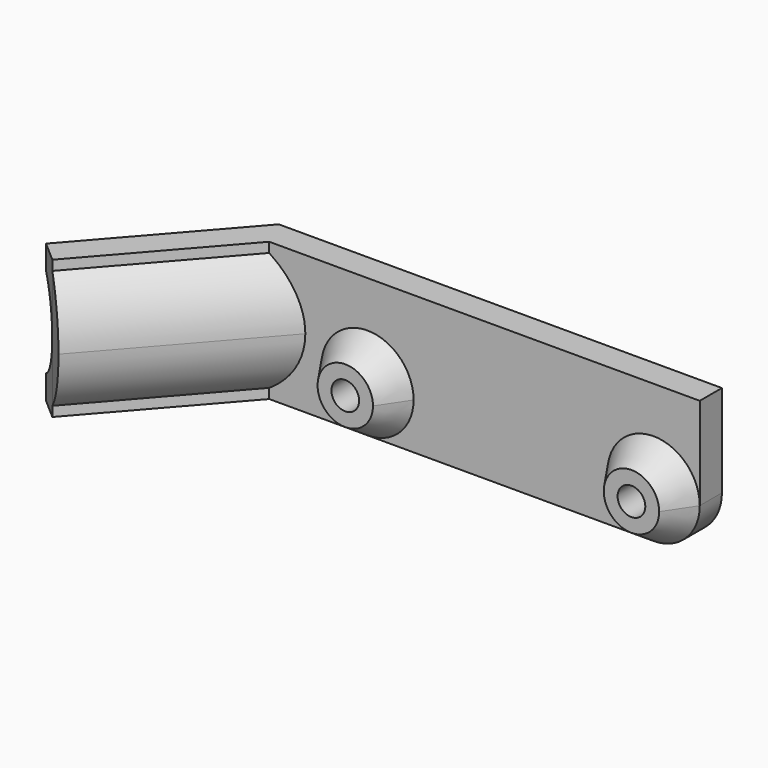
from build123d import *

# Parameters (mm, degrees)
F1_DEPTH   = 15
F3_DEPTH   = 22
F4_DEPTH   = 25
F6_D       = 3
F6_DEPTH   = 5
F6_TIP     = 0.9012909285
F7_DEPTH   = 3
F8_D       = 3
F8_DEPTH   = 5
F8_TIP     = 0.9012909285
F9_SIZE2   = 2.99999
F9_SIZE    = 1.99999
F9_2_SIZE2 = 2.99999
F9_2_SIZE  = 1.99999
F10_R      = 5


# Not quite as in the source:
# - a fillet or chamfer is up to 0.001 mm smaller than in the source, because OpenCascade refuses the exact size


with BuildPart() as f1:
    # F0 (on Top) → F1 (new body)
    with BuildSketch(Plane.XY):
        Polygon((-4.7512178265, 0), (41.8870657801, 0), (41.8870657801, 3), (-6.1129342199, 3), (-19.2796003392, -12.0545309891), (-17.0214206908, -14.029530907), align=None)
    extrude(amount=F1_DEPTH)

    # F2 (on face) → F3 (join)
    with BuildSketch(Plane(origin=(-14.3293936969, -16.3839729443, 0), x_dir=(0.7527265495, -0.658333306, 0), z_dir=(-0.658333306, -0.7527265495, 0))):
        with BuildLine():
            ThreePointArc((-0.6336620972, 7.5), (-1.4042700925, 11.0364529176), (-3.5763678003, 13.9316778603))
            Line((-3.5763678003, 13.9316778603), (-3.5763678003, 1.0683221397))
            ThreePointArc((-3.5763678003, 1.0683221397), (-1.4042700925, 3.9635470824), (-0.6336620972, 7.5))
        make_face()
    extrude(amount=-F3_DEPTH)

    # F2 (on face) → F4 (cut)
    with BuildSketch(Plane(origin=(-14.3293936969, -16.3839729443, 0), x_dir=(0.7527265495, -0.658333306, 0), z_dir=(-0.658333306, -0.7527265495, 0))):
        with BuildLine():
            ThreePointArc((-6.5763678003, 2.6306832225), (-4.4264804227, 4.6552784524), (-3.6336620972, 7.5))
            ThreePointArc((-3.6336620972, 7.5), (-4.4264804227, 10.3447215476), (-6.5763678003, 12.3693167775))
            Line((-6.5763678003, 12.3693167775), (-6.5763678003, 2.6306832225))
        make_face()
    extrude(amount=-F4_DEPTH, mode=Mode.SUBTRACT)

    # F6
    with Locations(Plane.XZ):
        with Locations((5.8870657801, 5), (36.8870657801, 5)):
            Hole(F6_D / 2, depth=F6_DEPTH)
            with Locations((0, 0, -(F6_DEPTH + F6_TIP / 2))):  # 118° drill point
                Cone(0, F6_D / 2, F6_TIP, mode=Mode.SUBTRACT)

    # F5 (on face) → F7 (join)
    with BuildSketch(Plane.XZ):
        with BuildLine():
            ThreePointArc((5.8870657801, 0), (9.422599686, 1.4644660941), (10.8870657801, 5))
            ThreePointArc((10.8870657801, 5), (2.3515318742, 8.5355339059), (5.8870657801, 0))
        make_face()
        with BuildLine():
            ThreePointArc((41.8870657801, 5), (33.3515318742, 8.5355339059), (36.8870657801, 0))
            ThreePointArc((36.8870657801, 0), (40.422599686, 1.4644660941), (41.8870657801, 5))
        make_face()
    extrude(amount=F7_DEPTH)

    # F8
    with Locations(Plane(origin=(0, 0, 0), x_dir=(1, 0, 0), z_dir=(0, 1, 0))):
        with Locations((5.8870657801, -5), (36.8870657801, -5)):
            Hole(F8_D / 2, depth=F8_DEPTH)
            with Locations((0, 0, -(F8_DEPTH + F8_TIP / 2))):  # 118° drill point
                Cone(0, F8_D / 2, F8_TIP, mode=Mode.SUBTRACT)

    # F9 (size 2 and 3 in the source; OpenCascade refuses exactly that, so slightly less here)
    f9_edges = [f1.edges().sort_by_distance(p)[0] for p in [
        (5.887066, -3, 10),
    ]]
    f9_side = f1.faces().sort_by_distance((5.887066, -3, 9.858579))[0]
    chamfer(f9_edges, length=F9_SIZE, length2=F9_SIZE2, reference=f9_side)

    # F9#2 (size 2 and 3 in the source; OpenCascade refuses exactly that, so slightly less here)
    f9_2_edges = [f1.edges().sort_by_distance(p)[0] for p in [
        (31.887066, -3, 5),
    ]]
    f9_2_side = f1.faces().sort_by_distance((32.028487, -3, 5))[0]
    chamfer(f9_2_edges, length=F9_2_SIZE, length2=F9_2_SIZE2, reference=f9_2_side)

    # F10
    f10_edges = [f1.edges().sort_by_distance(p)[0] for p in [
        (41.887066, 1.5, 0),
    ]]
    fillet(f10_edges, radius=F10_R)


solid = f1.part
